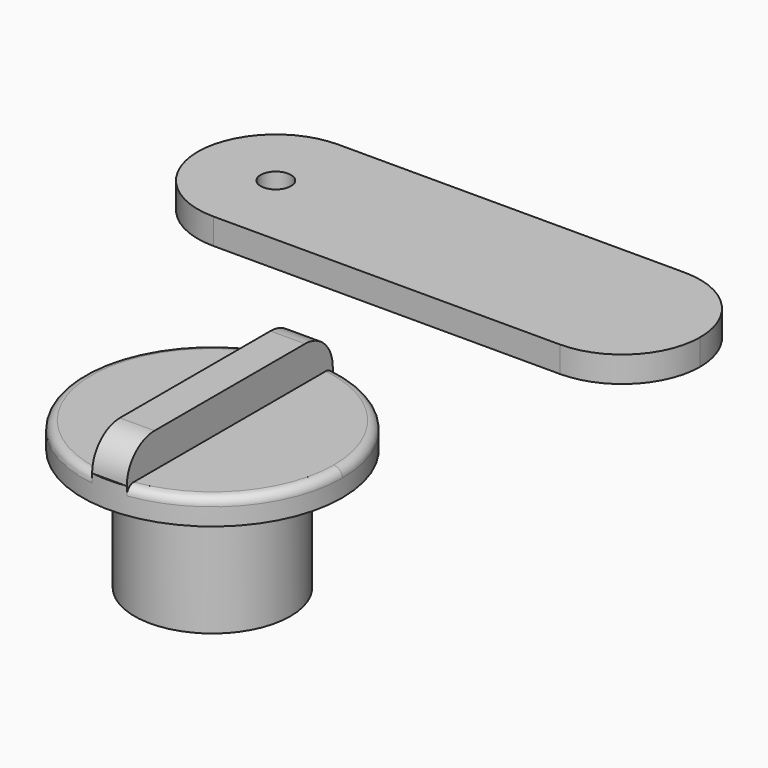
from build123d import *

# Parameters (mm, degrees)
F0_R         = 15
F1_DEPTH     = 3
F2_R         = 9
F3_DEPTH     = 14
F4_W         = 4
F4_H         = 29.7321374946
F5_DEPTH     = 4
F6_R         = 3.99999
F7_T4_ANGLE  = 164.6754886785
F7_T9_ANGLE  = 82.3377443392
F7_T14_ANGLE = 82.3377443392
F8_R         = 1.25
F9_DEPTH     = 7
F10_W        = 58
F10_H        = 18
F10_R        = 1.75
F11_DEPTH    = 3
F12_R        = 8.99999


# Not quite as in the source:
# - a fillet or chamfer that OpenCascade refuses, or shapes differently, is made with other operations: its cross-section is extruded or revolved along the edge and cut away or added
# - a fillet or chamfer is up to 0.001 mm smaller than in the source, because OpenCascade refuses the exact size


with BuildPart() as f1:
    # F0 (on Top) → F1 (new body)
    with BuildSketch(Plane.XY):
        Circle(F0_R)
    extrude(amount=F1_DEPTH)

    # F2 (on face) → F3 (join)
    with BuildSketch(Plane(origin=(0, 0, 0), x_dir=(1, 0, 0), z_dir=(0, 0, -1))):
        Circle(F2_R)
    extrude(amount=F3_DEPTH)

    # F4 (on face) → F5 (join)
    with BuildSketch(Plane.XY.offset(3)):
        Rectangle(F4_W, F4_H)
    extrude(amount=F5_DEPTH)

    # F6 (radius 4 in the source; OpenCascade refuses exactly that, so slightly less here)
    f6_edges = [f1.edges().sort_by_distance(p)[0] for p in [
        (0, 14.866069, 7),
        (0, -14.866069, 7),
    ]]
    fillet(f6_edges, radius=F6_R)

    # F7: fillet of radius 1 on 3 edges, made by hand


with BuildPart() as f7_tool2:
    # F7_s3 → F7_t4 (revolve)
    with BuildSketch(Plane(origin=(0, 0, 0), x_dir=(0, 0, 1), z_dir=(0.9910712498, 0.1333333333, 0))):
        with BuildLine():
            ThreePointArc((2, -15), (2.7071067812, -14.7071067812), (3, -14))
            Line((3, -14), (3, -15))
            Line((3, -15), (2, -15))
        make_face()
    revolve(axis=Axis((0, 0, 3), (0, 0, 1)), revolution_arc=F7_T4_ANGLE)

    split(bisect_by=Plane.YZ.offset(-2), keep=Keep.BOTTOM)


with BuildPart() as f1_1:
    add(f1.part)

    # F7_t1: cut F7_tool2
    add(f7_tool2.part, mode=Mode.SUBTRACT)


with BuildPart() as f7_tool7:
    # F7_s8 → F7_t9 (revolve)
    with BuildSketch(Plane(origin=(0, 0, 0), x_dir=(0, 0, 1), z_dir=(-0.9910712498, -0.1333333333, 0))):
        with BuildLine():
            ThreePointArc((3, -14), (2.7071067812, -14.7071067812), (2, -15))
            Line((2, -15), (3, -15))
            Line((3, -15), (3, -14))
        make_face()
    revolve(axis=Axis((0, 0, 3), (0, 0, 1)), revolution_arc=F7_T9_ANGLE)

    split(bisect_by=Plane.YZ.offset(2), keep=Keep.TOP)


with BuildPart() as f1_2:
    add(f1_1.part)

    # F7_t6: cut F7_tool7
    add(f7_tool7.part, mode=Mode.SUBTRACT)


with BuildPart() as f7_tool12:
    # F7_s13 → F7_t14 (revolve)
    with BuildSketch(Plane.XZ):
        with BuildLine():
            ThreePointArc((14, 3), (14.7071067812, 2.7071067812), (15, 2))
            Line((15, 2), (15, 3))
            Line((15, 3), (14, 3))
        make_face()
    revolve(axis=Axis((0, 0, 3), (0, 0, 1)), revolution_arc=F7_T14_ANGLE)

    split(bisect_by=Plane.YZ.offset(2), keep=Keep.TOP)


with BuildPart() as f1_3:
    add(f1_2.part)

    # F7_t11: cut F7_tool12
    add(f7_tool12.part, mode=Mode.SUBTRACT)

    # F8 (on face) → F9 (cut)
    with BuildSketch(Plane(origin=(0, 0, -14), x_dir=(1, 0, 0), z_dir=(0, 0, -1))):
        Circle(F8_R)
    extrude(amount=-F9_DEPTH, mode=Mode.SUBTRACT)


with BuildPart() as f11:
    # F10 (on Top) → F11 (new body)
    with BuildSketch(Plane.XY):
        with Locations((-4.7804481387, 40.116373837)):
            Rectangle(F10_W, F10_H)
        with Locations((-24.7804481387, 40.116373837)):
            Circle(F10_R, mode=Mode.SUBTRACT)
    extrude(amount=F11_DEPTH)

    # F12 (radius 9 in the source; OpenCascade refuses exactly that, so slightly less here)
    f12_edges = [f11.edges().sort_by_distance(p)[0] for p in [
        (-33.780448, 49.116374, 1.5),
        (-33.780448, 31.116374, 1.5),
        (24.219552, 49.116374, 1.5),
        (24.219552, 31.116374, 1.5),
    ]]
    fillet(f12_edges, radius=F12_R)


solid = Compound([f1_3.part, f11.part])
